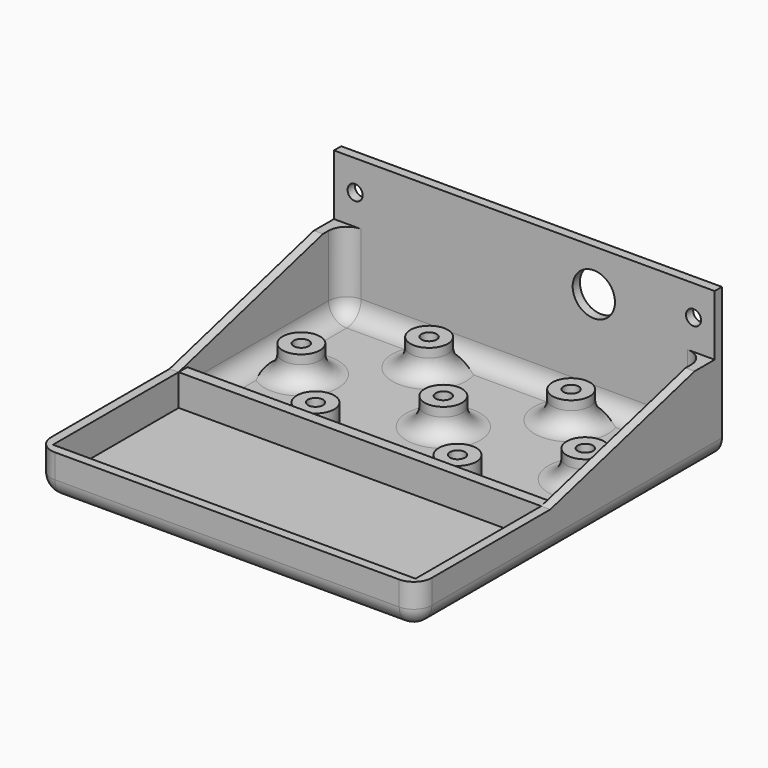
from build123d import *

# Parameters (mm, degrees)
F1_DEPTH      = 25
F0_W          = 60
F0_H          = 26
F0_H_2        = 32.2
F0_H_3        = 1.8
F2_DEPTH      = 1.8
F3_DEPTH      = 7
F4_R          = 3.1
F4_R_2        = 1.25
F5_DEPTH      = 6.3
F6_DEPTH      = 15
F7_DEPTH      = 7
F8_SIZE2      = 29.856396
F8_SIZE       = 7.99999
F9_SIZE2      = 29.856396
F9_SIZE       = 7.99999
F10_R         = 1.25
F10_R_2       = 3.5
F11_DEPTH     = 31.501
F12_T1_DEPTH  = 54
F12_T3_DEPTH  = 60
F12_T5_DEPTH  = 10.2
F12_S9_W      = 3.06
F12_S9_H      = 3.06
F12_T10_DEPTH = 3.06
F12_S15_W     = 3.06
F12_S15_H     = 3.06
F12_T16_DEPTH = 3.06
F12_T32_DEPTH = 75
F12_S35_R     = 1.25
F12_T36_DEPTH = 39
F12_S37_R     = 1.25
F12_T38_DEPTH = 39
F12_T42_DEPTH = 36.7
F12_T47_DEPTH = 36.7
F12_T49_DEPTH = 11.5
F12_T51_DEPTH = 57
F12_T53_DEPTH = 67.5
F12_S57_W     = 3.06
F12_S57_H     = 3.06
F12_T58_DEPTH = 3.06
F12_S63_W     = 3.06
F12_S63_H     = 3.06
F12_T64_DEPTH = 3.06


# Not quite as in the source:
# - a fillet or chamfer that OpenCascade refuses, or shapes differently, is made with other operations: its cross-section is extruded or revolved along the edge and cut away or added
# - a fillet or chamfer is up to 0.001 mm smaller than in the source, because OpenCascade refuses the exact size


with BuildPart() as f1:
    # F0 (on Top) → F1 (new body)
    with BuildSketch(Plane.XY):
        Polygon((-30, 30), (30, 30), (31.5, 30), (31.5, 31.5), (0, 31.5), (-31.5, 31.5), (-31.5, 30), align=None)
    extrude(amount=F1_DEPTH)

    # F0 (on Top) → F2 (join)
    with BuildSketch(Plane.XY):
        with Locations((0, -17)):
            Rectangle(F0_W, F0_H)
        Polygon((30, -4), (30, -30), (-30, -30), (-30, -4), (-31.5, -4), (-31.5, -5), (-31.5, -31.5), (-4.0078373849, -31.5), (31.5, -31.5), (31.5, -4), align=None)
        with Locations((0, 13.9)):
            Rectangle(F0_W, F0_H_2)
        with Locations((0, -3.1)):
            Rectangle(F0_W, F0_H_3)
    extrude(amount=F2_DEPTH)

    # F0 (on Top) → F3 (join)
    with BuildSketch(Plane.XY):
        with Locations((0, -3.1)):
            Rectangle(F0_W, F0_H_3)
    extrude(amount=F3_DEPTH)

    # F4 (on Top) → F5 (join)
    with BuildSketch(Plane.XY):
        with Locations((23.5, 13.25)):
            Circle(F4_R)
        with Locations((23.5, 13.25)):
            Circle(F4_R_2, mode=Mode.SUBTRACT)
        with Locations((11.75, 1.5)):
            Circle(F4_R)
        with Locations((11.75, 1.5)):
            Circle(F4_R_2, mode=Mode.SUBTRACT)
        with Locations((11.75, 25)):
            Circle(F4_R)
        with Locations((11.75, 25)):
            Circle(F4_R_2, mode=Mode.SUBTRACT)
        with Locations((0, 13.25)):
            Circle(F4_R)
        with Locations((0, 13.25)):
            Circle(F4_R_2, mode=Mode.SUBTRACT)
        with Locations((-11.75, 25)):
            Circle(F4_R)
        with Locations((-11.75, 25)):
            Circle(F4_R_2, mode=Mode.SUBTRACT)
        with Locations((-11.75, 1.5)):
            Circle(F4_R)
        with Locations((-11.75, 1.5)):
            Circle(F4_R_2, mode=Mode.SUBTRACT)
        with Locations((-23.5, 13.25)):
            Circle(F4_R)
        with Locations((-23.5, 13.25)):
            Circle(F4_R_2, mode=Mode.SUBTRACT)
    extrude(amount=F5_DEPTH)

    # F0 (on Top) → F6 (join)
    with BuildSketch(Plane.XY):
        Polygon((-31.5, -4), (-30, -4), (-30, -2.2), (-30, 30), (-31.5, 30), (-31.5, 5), align=None)
        Polygon((30, -2.2), (30, -4), (31.5, -4), (31.5, 30), (30, 30), align=None)
    extrude(amount=F6_DEPTH)

    # F0 (on Top) → F7 (join)
    with BuildSketch(Plane.XY):
        Polygon((30, -4), (30, -30), (-30, -30), (-30, -4), (-31.5, -4), (-31.5, -5), (-31.5, -31.5), (-4.0078373849, -31.5), (31.5, -31.5), (31.5, -4), align=None)
    extrude(amount=F7_DEPTH)

    # F8 (size 8 and 29.8564064606 in the source; OpenCascade refuses exactly that, so slightly less here)
    f8_edges = [f1.edges().sort_by_distance(p)[0] for p in [
        (-30.75, -4, 15),
    ]]
    f8_side = f1.faces().sort_by_distance((-30.75, -4, 11))[0]
    chamfer(f8_edges, length=F8_SIZE, length2=F8_SIZE2, reference=f8_side)

    # F9 (size 8 and 29.8564064606 in the source; OpenCascade refuses exactly that, so slightly less here)
    f9_edges = [f1.edges().sort_by_distance(p)[0] for p in [
        (30.75, -4, 15),
    ]]
    f9_side = f1.faces().sort_by_distance((30.75, -4, 11))[0]
    chamfer(f9_edges, length=F9_SIZE, length2=F9_SIZE2, reference=f9_side)

    # F10 (on Front) → F11 (cut, through all)
    with BuildSketch(Plane.XZ):
        with Locations((28, 20)):
            Circle(F10_R)
        with Locations((-28, 20)):
            Circle(F10_R)
        with Locations((11.5, 18.0163495243)):
            Circle(F10_R_2)
    extrude(amount=-F11_DEPTH, mode=Mode.SUBTRACT)

    # F12: fillet of radius 3 on 17 edges, made by hand

    # F12_s2 → F12_t1 (join)
    with BuildSketch(Plane.YZ.offset(-27)):
        with BuildLine():
            ThreePointArc((30, 4.8), (29.1213203436, 2.6786796564), (27, 1.8))
            Line((27, 1.8), (30, 1.8))
            Line((30, 1.8), (30, 4.8))
        make_face()
    extrude(amount=F12_T1_DEPTH)

    # F12_s4 → F12_t3 (join)
    with BuildSketch(Plane.YZ.offset(-30)):
        with BuildLine():
            ThreePointArc((-30, 4.8), (-29.1213203436, 2.6786796564), (-27, 1.8))
            Line((-27, 1.8), (-30, 1.8))
            Line((-30, 1.8), (-30, 4.8))
        make_face()
    extrude(amount=F12_T3_DEPTH)

    # F12_s6 → F12_t5 (join)
    with BuildSketch(Plane.XY.offset(4.8)):
        with BuildLine():
            ThreePointArc((30, 27), (29.1213203436, 29.1213203436), (27, 30))
            Line((27, 30), (30, 30))
            Line((30, 30), (30, 27))
        make_face()
        with BuildLine():
            ThreePointArc((-27, 30), (-29.1213203436, 29.1213203436), (-30, 27))
            Line((-30, 27), (-30, 30))
            Line((-30, 30), (-27, 30))
        make_face()
    extrude(amount=F12_T5_DEPTH)


with BuildPart() as f12_tool8:
    # F12_s9 → F12_t10 (new body)
    with BuildSketch(Plane.YZ.offset(27)):
        with Locations((28.53, 3.27)):
            Rectangle(F12_S9_W, F12_S9_H)
    extrude(amount=F12_T10_DEPTH)

    # F12_s11 → F12_t12 (revolve, cut)
    with BuildSketch(Plane(origin=(27, 27, 4.8), x_dir=(0, -0.7071067812, 0.7071067812), z_dir=(0, 0.7071067812, 0.7071067812))):
        with BuildLine():
            ThreePointArc((0, -3), (3, 0), (0, 3))
            Line((0, 3), (0, -3))
        make_face()
    revolve(axis=Axis((27, 27, 4.8), (1, 0, 0)), mode=Mode.SUBTRACT)


with BuildPart() as f1_1:
    add(f1.part)

    # F12_t7: union F12_tool8
    add(f12_tool8.part)


with BuildPart() as f12_tool14:
    # F12_s15 → F12_t16 (new body)
    with BuildSketch(Plane.YZ.offset(-27)):
        with Locations((28.53, 3.27)):
            Rectangle(F12_S15_W, F12_S15_H)
    extrude(amount=-F12_T16_DEPTH)

    # F12_s17 → F12_t18 (revolve, cut)
    with BuildSketch(Plane(origin=(-27, 27, 4.8), x_dir=(0, -0.7071067812, 0.7071067812), z_dir=(0, -0.7071067812, -0.7071067812))):
        with BuildLine():
            ThreePointArc((0, -3), (3, 0), (0, 3))
            Line((0, 3), (0, -3))
        make_face()
    revolve(axis=Axis((-27, 27, 4.8), (-1, 0, 0)), mode=Mode.SUBTRACT)


with BuildPart() as f1_2:
    add(f1_1.part)

    # F12_t13: union F12_tool14
    add(f12_tool14.part)

    # F12_s19 → F12_t20 (revolve)
    with BuildSketch(Plane.XZ.offset(-25)):
        with BuildLine():
            ThreePointArc((-5.65, 1.8), (-7.7713203436, 2.6786796564), (-8.65, 4.8))
            Line((-8.65, 4.8), (-8.65, 1.8))
            Line((-8.65, 1.8), (-5.65, 1.8))
        make_face()
    revolve(axis=Axis((-11.75, 25, 1.8), (0, 0, -1)))

    # F12_s21 → F12_t22 (revolve)
    with BuildSketch(Plane.XZ.offset(-13.25)):
        with BuildLine():
            ThreePointArc((-17.4, 1.8), (-19.5213203436, 2.6786796564), (-20.4, 4.8))
            Line((-20.4, 4.8), (-20.4, 1.8))
            Line((-20.4, 1.8), (-17.4, 1.8))
        make_face()
    revolve(axis=Axis((-23.5, 13.25, 1.8), (0, 0, -1)))

    # F12_s23 → F12_t24 (revolve)
    with BuildSketch(Plane.XZ.offset(-13.25)):
        with BuildLine():
            ThreePointArc((6.1, 1.8), (3.9786796564, 2.6786796564), (3.1, 4.8))
            Line((3.1, 4.8), (3.1, 1.8))
            Line((3.1, 1.8), (6.1, 1.8))
        make_face()
    revolve(axis=Axis((0, 13.25, 1.8), (0, 0, -1)))

    # F12_s25 → F12_t26 (revolve)
    with BuildSketch(Plane.XZ.offset(-25)):
        with BuildLine():
            ThreePointArc((17.85, 1.8), (15.7286796564, 2.6786796564), (14.85, 4.8))
            Line((14.85, 4.8), (14.85, 1.8))
            Line((14.85, 1.8), (17.85, 1.8))
        make_face()
    revolve(axis=Axis((11.75, 25, 1.8), (0, 0, -1)))

    # F12_s27 → F12_t28 (revolve)
    with BuildSketch(Plane.XZ.offset(-13.25)):
        with BuildLine():
            ThreePointArc((29.6, 1.8), (27.4786796564, 2.6786796564), (26.6, 4.8))
            Line((26.6, 4.8), (26.6, 1.8))
            Line((26.6, 1.8), (29.6, 1.8))
        make_face()
    revolve(axis=Axis((23.5, 13.25, 1.8), (0, 0, -1)))


with BuildPart() as f12_tool30:
    # F12_s31 → F12_t32 (new body)
    with BuildSketch(Plane.YZ.offset(-37.5)):
        with BuildLine():
            ThreePointArc((-2.2, 4.8), (-1.3213203436, 2.6786796564), (0.8, 1.8))
            Line((0.8, 1.8), (-2.2, 1.8))
            Line((-2.2, 1.8), (-2.2, 4.8))
        make_face()
    extrude(amount=F12_T32_DEPTH)

    split(bisect_by=Plane.YZ.offset(31.5), keep=Keep.BOTTOM)

    split(bisect_by=Plane.YZ.offset(-31.5), keep=Keep.TOP)

    # F12_s35 → F12_t36 (cut, symmetric)
    with BuildSketch(Plane.XY.offset(3.3)):
        with Locations((-11.75, 1.5)):
            Circle(F12_S35_R)
    extrude(amount=F12_T36_DEPTH, both=True, mode=Mode.SUBTRACT)

    # F12_s37 → F12_t38 (cut, symmetric)
    with BuildSketch(Plane.XY.offset(3.3)):
        with Locations((11.75, 1.5)):
            Circle(F12_S37_R)
    extrude(amount=F12_T38_DEPTH, both=True, mode=Mode.SUBTRACT)


with BuildPart() as f1_3:
    add(f1_2.part)

    # F12_t29: union F12_tool30
    add(f12_tool30.part)


with BuildPart() as f12_tool40:
    # F12_s41 → F12_t42 (new body)
    with BuildSketch(Plane.XZ.offset(-27)):
        with BuildLine():
            ThreePointArc((-27, 1.8), (-29.1213203436, 2.6786796564), (-30, 4.8))
            Line((-30, 4.8), (-30, 1.8))
            Line((-30, 1.8), (-27, 1.8))
        make_face()
    extrude(amount=F12_T42_DEPTH)

    split(bisect_by=Plane.XZ.offset(4), keep=Keep.BOTTOM)


with BuildPart() as f1_4:
    add(f1_3.part)

    # F12_t39: union F12_tool40
    add(f12_tool40.part)


with BuildPart() as f12_tool45:
    # F12_s46 → F12_t47 (new body)
    with BuildSketch(Plane.XZ.offset(9.7)):
        with BuildLine():
            ThreePointArc((30, 4.8), (29.1213203436, 2.6786796564), (27, 1.8))
            Line((27, 1.8), (30, 1.8))
            Line((30, 1.8), (30, 4.8))
        make_face()
    extrude(amount=-F12_T47_DEPTH)

    split(bisect_by=Plane.XZ.offset(4), keep=Keep.BOTTOM)


with BuildPart() as f1_5:
    add(f1_4.part)

    # F12_t44: union F12_tool45
    add(f12_tool45.part)

    # F12_s50 → F12_t49 (cut)
    with BuildSketch(Plane.XY.offset(3)):
        with BuildLine():
            ThreePointArc((-28.5, -31.5), (-30.6213203436, -30.6213203436), (-31.5, -28.5))
            Line((-31.5, -28.5), (-31.5, -31.5))
            Line((-31.5, -31.5), (-28.5, -31.5))
        make_face()
        with BuildLine():
            ThreePointArc((28.5, -31.5), (30.6213203436, -30.6213203436), (31.5, -28.5))
            Line((31.5, -28.5), (31.5, -31.5))
            Line((31.5, -31.5), (28.5, -31.5))
        make_face()
    extrude(amount=F12_T49_DEPTH, mode=Mode.SUBTRACT)

    # F12_s52 → F12_t51 (cut)
    with BuildSketch(Plane.YZ.offset(-28.5)):
        with BuildLine():
            ThreePointArc((-31.5, 3), (-30.6213203436, 0.8786796564), (-28.5, 0))
            Line((-28.5, 0), (-31.5, 0))
            Line((-31.5, 0), (-31.5, 3))
        make_face()
    extrude(amount=F12_T51_DEPTH, mode=Mode.SUBTRACT)

    # F12_s54 → F12_t53 (cut)
    with BuildSketch(Plane.XZ.offset(-39)):
        with BuildLine():
            ThreePointArc((28.5, 0), (30.6213203436, 0.8786796564), (31.5, 3))
            Line((31.5, 3), (31.5, 0))
            Line((31.5, 0), (28.5, 0))
        make_face()
        with BuildLine():
            ThreePointArc((-28.5, 0), (-30.6213203436, 0.8786796564), (-31.5, 3))
            Line((-31.5, 3), (-31.5, 0))
            Line((-31.5, 0), (-28.5, 0))
        make_face()
    extrude(amount=F12_T53_DEPTH, mode=Mode.SUBTRACT)


with BuildPart() as f12_tool56:
    # F12_s57 → F12_t58 (new body)
    with BuildSketch(Plane.XZ.offset(28.5)):
        with Locations((-30.03, 1.47)):
            Rectangle(F12_S57_W, F12_S57_H)
    extrude(amount=F12_T58_DEPTH)

    # F12_s59 → F12_t60 (revolve, cut)
    with BuildSketch(Plane(origin=(-28.5, -28.5, 3), x_dir=(0.7071067812, 0, 0.7071067812), z_dir=(0.7071067812, 0, -0.7071067812))):
        with BuildLine():
            ThreePointArc((0, -3), (3, 0), (0, 3))
            Line((0, 3), (0, -3))
        make_face()
    revolve(axis=Axis((-28.5, -28.5, 3), (0, -1, 0)), mode=Mode.SUBTRACT)


with BuildPart() as f1_6:
    add(f1_5.part)

    # F12_t55: cut F12_tool56
    add(f12_tool56.part, mode=Mode.SUBTRACT)


with BuildPart() as f12_tool62:
    # F12_s63 → F12_t64 (new body)
    with BuildSketch(Plane.XZ.offset(28.5)):
        with Locations((30.03, 1.47)):
            Rectangle(F12_S63_W, F12_S63_H)
    extrude(amount=F12_T64_DEPTH)

    # F12_s65 → F12_t66 (revolve, cut)
    with BuildSketch(Plane(origin=(28.5, -28.5, 3), x_dir=(-0.7071067812, 0, 0.7071067812), z_dir=(0.7071067812, 0, 0.7071067812))):
        with BuildLine():
            ThreePointArc((0, -3), (3, 0), (0, 3))
            Line((0, 3), (0, -3))
        make_face()
    revolve(axis=Axis((28.5, -28.5, 3), (0, -1, 0)), mode=Mode.SUBTRACT)


with BuildPart() as f1_7:
    add(f1_6.part)

    # F12_t61: cut F12_tool62
    add(f12_tool62.part, mode=Mode.SUBTRACT)


solid = f1_7.part
